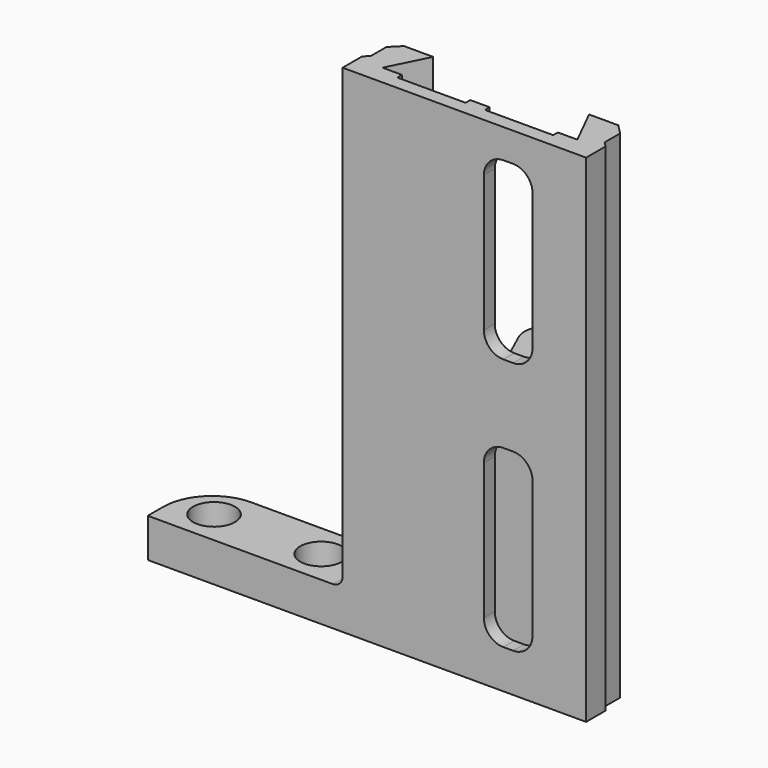
from build123d import *

# Parameters (mm, degrees)
F1_DEPTH      = 50
F0_W          = 7
F0_H          = 0.6
F2_DEPTH      = 1
F3_T4_DEPTH   = 51
F3_T9_DEPTH   = 51
F3_T11_DEPTH  = 56.1433659759
F5_DEPTH      = 25
F6_DEPTH      = 25
F0_R          = 2.15
F7_DEPTH      = 3
F7_DEPTH_BACK = 1
F8_R          = 1
F9_T1_DEPTH   = 18.9997500167
F9_T3_DEPTH   = 28.9992500113


# Not quite as in the source:
# - a fillet or chamfer that OpenCascade refuses, or shapes differently, is made with other operations: its cross-section is extruded or revolved along the edge and cut away or added


with BuildPart() as f1:
    # F0 (on Top) → F1 (new body)
    with BuildSketch(Plane.XY):
        Polygon((2, 0), (0, 0), (-2, 0), (-0.5, -3), (0, -4), (2, -4), align=None)
        Polygon((-19.5, -3), (-18, 0), (-20, 0), (-22, 0), (-22, -4), (-20, -4), align=None)
        Polygon((2.5, -4), (2, -4), (0, -4), (-0.5, -4), (-2, -4), (-2, -4.6), (-9, -4.6), (-9, -4), (-11, -4), (-11, -4.6), (-18, -4.6), (-18, -4), (-19.5, -4), (-20, -4), (-22, -4), (-22.5, -4), (-22.5, -6), (2.5, -6), align=None)
    extrude(amount=F1_DEPTH)

    # F0 (on Top) + F1_face (on face) → F2 (join)
    with BuildSketch(Plane.XY):
        Polygon((2, 0), (0, 0), (-2, 0), (-0.5, -3), (0, -4), (2, -4), align=None)
        Polygon((-0.5, -3), (-2, 0), (-18, 0), (-19.5, -3), (-19.5, -4), (-18, -4), (-11, -4), (-9, -4), (-2, -4), (-0.5, -4), align=None)
        Polygon((0, -4), (-0.5, -3), (-0.5, -4), align=None)
        Polygon((-19.5, -4), (-19.5, -3), (-20, -4), align=None)
        with Locations((-5.5, -4.3)):
            Rectangle(F0_W, F0_H)
        with Locations((-14.5, -4.3)):
            Rectangle(F0_W, F0_H)
    with BuildSketch(Plane(origin=(-10, -3.9107723577, 0), x_dir=(1, 0, 0), z_dir=(0, 0, -1))):
        Polygon((8, -3.9107723577), (12, -3.9107723577), (12, 0.0892276423), (12.5, 0.0892276423), (12.5, 2.0892276423), (-12.5, 2.0892276423), (-12.5, 0.0892276423), (-12, 0.0892276423), (-12, -3.9107723577), (-8, -3.9107723577), (-10, 0.0892276423), (-8, 0.0892276423), (-8, 0.6892276423), (-1, 0.6892276423), (-1, 0.0892276423), (1, 0.0892276423), (1, 0.6892276423), (8, 0.6892276423), (8, 0.0892276423), (10, 0.0892276423), align=None)
    extrude(amount=-F2_DEPTH, dir=(0, 0, 1))

    # F3: chamfer of 1 on 4 edges, made by hand


with BuildPart() as f3_tool2:
    # F3_s3 → F3_t4 (new body)
    with BuildSketch(Plane.XY.offset(-1)):
        Polygon((-23, -4), (-22, -3), (-22, -4), align=None)
    extrude(amount=F3_T4_DEPTH)

    split(bisect_by=Plane.YZ.offset(-22.5), keep=Keep.TOP)


with BuildPart() as f1_1:
    add(f1.part)

    # F3_t1: union F3_tool2
    add(f3_tool2.part)


with BuildPart() as f3_tool7:
    # F3_s8 → F3_t9 (new body)
    with BuildSketch(Plane.XY.offset(50)):
        Polygon((3, -4), (2, -3), (2, -4), align=None)
    extrude(amount=-F3_T9_DEPTH)

    split(bisect_by=Plane.YZ.offset(2.5), keep=Keep.BOTTOM)


with BuildPart() as f1_2:
    add(f1_1.part)

    # F3_t6: union F3_tool7
    add(f3_tool7.part)

    # F3_s12 → F3_t11 (cut)
    with BuildSketch(Plane.XY.offset(-3.571682988)):
        Polygon((-21, 0), (-22, -1), (-22, 0), align=None)
        Polygon((1, 0), (2, -1), (2, 0), align=None)
    extrude(amount=F3_T11_DEPTH, mode=Mode.SUBTRACT)

    # F4 (on face) → F5 (cut)
    with BuildSketch(Plane(origin=(0, -4, 0), x_dir=(-1, 0, 0), z_dir=(0, 1, 0))):
        with BuildLine():
            ThreePointArc((8, 45), (7.4142135624, 46.4142135624), (6, 47))
            Line((6, 47), (5, 47))
            ThreePointArc((5, 47), (3.5857864376, 46.4142135624), (3, 45))
            Line((3, 45), (3, 31))
            ThreePointArc((3, 31), (3.5857864376, 29.5857864376), (5, 29))
            Line((5, 29), (6, 29))
            ThreePointArc((6, 29), (7.4142135624, 29.5857864376), (8, 31))
            Line((8, 31), (8, 45))
        make_face()
        with BuildLine():
            ThreePointArc((8, 19), (7.4142135624, 20.4142135624), (6, 21))
            Line((6, 21), (5, 21))
            ThreePointArc((5, 21), (3.5857864376, 20.4142135624), (3, 19))
            Line((3, 19), (3, 5))
            ThreePointArc((3, 5), (3.5857864376, 3.5857864376), (5, 3))
            Line((5, 3), (6, 3))
            ThreePointArc((6, 3), (7.4142135624, 3.5857864376), (8, 5))
            Line((8, 5), (8, 19))
        make_face()
    extrude(amount=-F5_DEPTH, mode=Mode.SUBTRACT)

    # F0 (on Top) → F7 (join, two sides)
    with BuildSketch(Plane.XY) as f7_sk:
        Polygon((-22, -4), (-22, 0), (-22, 1), (-42.5, 1), (-42.5, -6), (-22.5, -6), (-22.5, -4), align=None)
        with Locations((-38.5, -2.5)):
            Circle(F0_R, mode=Mode.SUBTRACT)
        with Locations((-27.5, -2.5)):
            Circle(F0_R, mode=Mode.SUBTRACT)
        Polygon((-19.5, -3), (-18, 0), (-20, 0), (-22, 0), (-22, -4), (-20, -4), align=None)
    extrude(amount=F7_DEPTH)
    extrude(f7_sk.sketch, amount=-F7_DEPTH_BACK)

    # F8
    f8_edges = [f1_2.edges().sort_by_distance(p)[0] for p in [
        (-22.5, -4.75, 3),
        (-22.25, -3.25, 3),
        (-22, -2, 3),
        (-21.5, -0.5, 3),
    ]]
    fillet(f8_edges, radius=F8_R)

    # F9: fillet of radius 5 on 2 edges, made by hand

    # F9_s2 → F9_t1 (cut)
    with BuildSketch(Plane.XY.offset(-8.4998750083)):
        with BuildLine():
            ThreePointArc((-21.9999099988, 0.0001199991), (-23.4187874519, 0.7435585843), (-24.9999499996, 1.00015))
            Line((-24.9999499996, 1.00015), (-24.9999499996, 1.10015))
            ThreePointArc((-24.9999499996, 1.10015), (-23.4999749998, 1.1), (-22, 1.1))
            Line((-22, 1.1), (-21.9, 1))
            ThreePointArc((-21.9, 1), (-21.9, 0.5000599995), (-21.9399091988, 0.0801193991))
            Line((-21.9399091988, 0.0801193991), (-21.9999099988, 0.0001199991))
        make_face()
    extrude(amount=F9_T1_DEPTH, mode=Mode.SUBTRACT)

    # F9_s4 → F9_t3 (cut)
    with BuildSketch(Plane.XY.offset(-13.4996250056)):
        with BuildLine():
            ThreePointArc((-37.50015, 1.00015), (-41.0356839059, -0.4643160941), (-42.50015, -3.99985))
            Line((-42.50015, -3.99985), (-42.60015, -3.99985))
            ThreePointArc((-42.60015, -3.99985), (-42.6, -1.499925), (-42.6, 1))
            Line((-42.6, 1), (-42.5, 1.1))
            ThreePointArc((-42.5, 1.1), (-40.000075, 1.1), (-37.50015, 1.10015))
            Line((-37.50015, 1.10015), (-37.50015, 1.00015))
        make_face()
    extrude(amount=F9_T3_DEPTH, mode=Mode.SUBTRACT)


with BuildPart() as f6:
    # F0 (on Top) → F6 (new body)
    with BuildSketch(Plane.XY):
        with BuildLine():
            ThreePointArc((-12.2765340768, 3.8128364101), (-10, 2.3459833488), (-7.7234659232, 3.8128364101))
            ThreePointArc((-7.7234659232, 3.8128364101), (-7.5565050448, 4.317464282), (-7.5, 4.8459833488))
            ThreePointArc((-7.5, 4.8459833488), (-10.5285190668, 7.289478304), (-12.2765340768, 3.8128364101))
        make_face()
        with BuildLine():
            Line((-18, 0), (-2, 0))
            Line((-2, 0), (-2, 1))
            Line((-2, 1), (-8.2240074562, 1))
            ThreePointArc((-8.2240074562, 1), (-8.6443137099, 1.2291815127), (-8.6793142716, 1.7066293877))
            Line((-8.6793142716, 1.7066293877), (-7.7234659232, 3.8128364101))
            ThreePointArc((-7.7234659232, 3.8128364101), (-10, 2.3459833488), (-12.2765340768, 3.8128364101))
            Line((-12.2765340768, 3.8128364101), (-11.3206857284, 1.7066293877))
            ThreePointArc((-11.3206857284, 1.7066293877), (-11.3556862901, 1.2291815127), (-11.7759925438, 1))
            Line((-11.7759925438, 1), (-18, 1))
            Line((-18, 1), (-18, 0))
        make_face()
        Polygon((-0.5, -3), (-2, 0), (-18, 0), (-19.5, -3), (-19.5, -4), (-18, -4), (-11, -4), (-9, -4), (-2, -4), (-0.5, -4), align=None)
    extrude(amount=F6_DEPTH)


solid = Compound([f1_2.part, f6.part])
